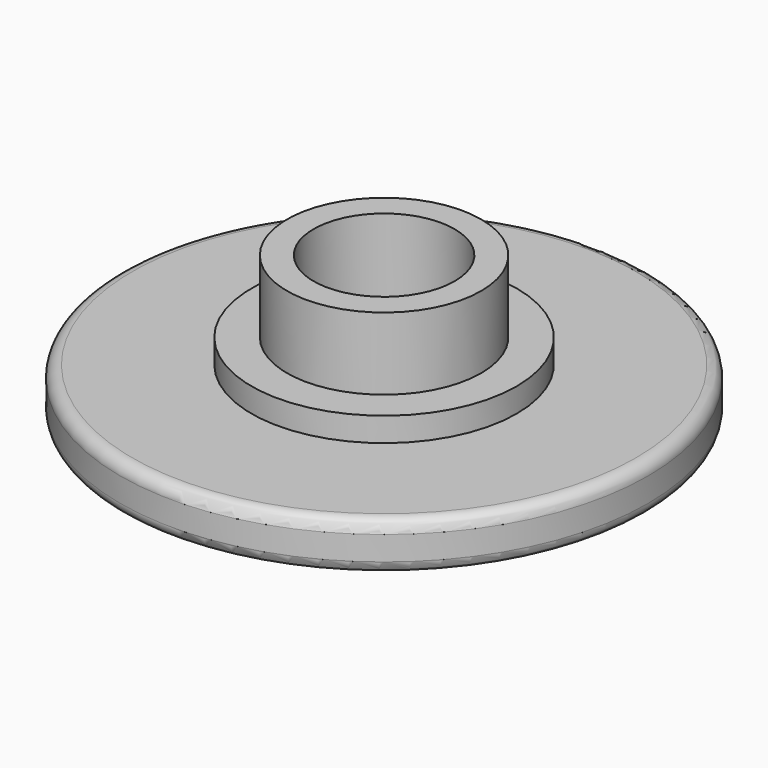
from build123d import *

# Parameters (mm, degrees)
F0_R         = 10.95
F0_R_2       = 0.069
F3_DEPTH     = 2
F1_R         = 5.5
F4_DEPTH     = 3
F2_R         = 4.025
F5_DEPTH     = 6
F6_R         = 0.5
F7_R         = 2.9249999207
F8_DEPTH     = 4
F9_TEXT_SIZE = 8.878378301
F10_DEPTH    = 1


# Not quite as in the source:
# - Text() gives the source's letters only with a copy of the font that has no kerning and outlines rounded to 1/6400 em; it was checked with that copy


with BuildPart() as f3:
    # F0 (on Top) → F3 (new body)
    with BuildSketch(Plane.XY):
        Circle(F0_R)
        Circle(F0_R_2, mode=Mode.SUBTRACT)
    extrude(amount=F3_DEPTH)

    # F1 (on Top) → F4 (join)
    with BuildSketch(Plane.XY):
        Circle(F1_R)
    extrude(amount=F4_DEPTH)

    # F2 (on Top) → F5 (join)
    with BuildSketch(Plane.XY):
        Circle(F2_R)
    extrude(amount=F5_DEPTH)

    # F6
    f6_edges = [f3.edges().sort_by_distance(p)[0] for p in [
        (10.95, 0, 1),
        (-10.95, 0, 0),
        (-10.95, 0, 2),
    ]]
    fillet(f6_edges, radius=F6_R)

    # F7 (on face) → F8 (cut)
    with BuildSketch(Plane.XY.offset(6)):
        Circle(F7_R)
    extrude(amount=-F8_DEPTH, mode=Mode.SUBTRACT)

    # F9 (on face) → F10 (cut)
    with BuildSketch(Plane(origin=(0, 0, 0), x_dir=(1, 0, 0), z_dir=(0, 0, -1))):
        with Locations((-9.7695351578, -3.1253886409)):
            Text('POLI', F9_TEXT_SIZE, font='Open Sans', text_align=(TextAlign.LEFT, TextAlign.BOTTOM))
    extrude(amount=-F10_DEPTH, mode=Mode.SUBTRACT)


solid = f3.part
